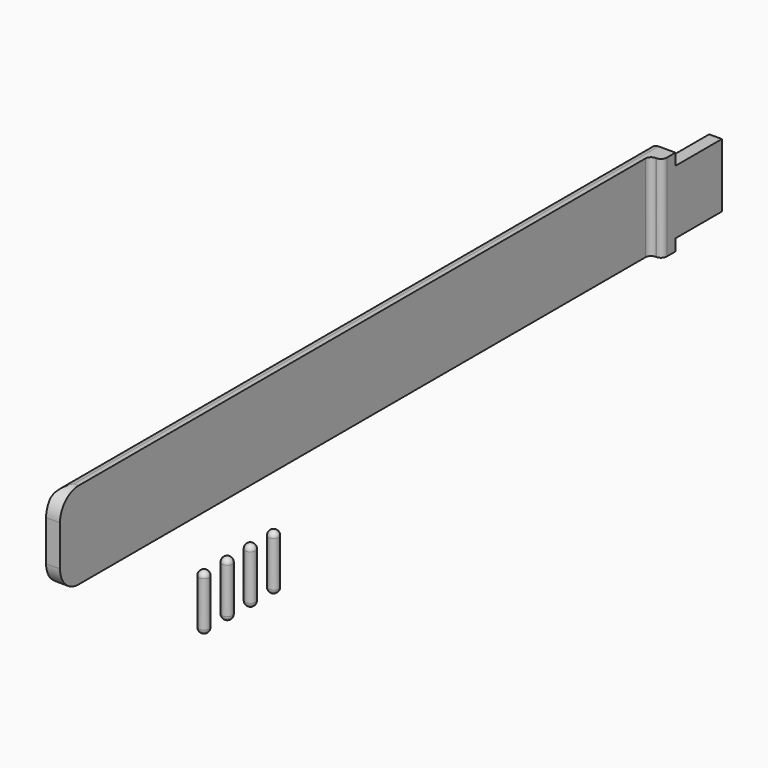
from build123d import *

# Parameters (mm, degrees)
F1_DEPTH    = 19.05
F2_T1_DEPTH = 28.448
F3_T1_DEPTH = 28.448
F4_R        = 1.27
F5_T1_DEPTH = 170.18
F6_W        = 12.7
F6_H        = 2.54
F7_DEPTH    = 25.4
F8_W        = 12.7
F8_H        = 2.54
F9_DEPTH    = 25.4
F10_R       = 1.143
F11_DEPTH   = 12.192
F12_R       = 1.143
F12_2_R     = 1.143
F12_3_R     = 1.143
F12_4_R     = 1.143


# Not quite as in the source:
# - a fillet or chamfer that OpenCascade refuses, or shapes differently, is made with other operations: its cross-section is extruded or revolved along the edge and cut away or added


with BuildPart() as f1:
    # F0 (on Top) → F1 (new body)
    with BuildSketch(Plane.XY):
        Polygon((0, 165.1), (0, 0), (3.048, 0), (3.048, 161.4486724138), (5.715, 161.4486724138), (5.715, 177.8), (2.921, 177.8), (2.921, 165.1), align=None)
    extrude(amount=F1_DEPTH)

    # F2: fillet of radius 5.08 on 1 edges, made by hand

    # F2_s2 → F2_t1 (cut)
    with BuildSketch(Plane.YZ.offset(-12.7)):
        with BuildLine():
            ThreePointArc((0, 13.97), (1.4878975516, 17.5621024484), (5.08, 19.05))
            Line((5.08, 19.05), (0, 19.05))
            Line((0, 19.05), (0, 13.97))
        make_face()
    extrude(amount=F2_T1_DEPTH, mode=Mode.SUBTRACT)

    # F3: fillet of radius 5.08 on 1 edges, made by hand

    # F3_s2 → F3_t1 (cut)
    with BuildSketch(Plane.YZ.offset(-12.7)):
        with BuildLine():
            ThreePointArc((5.08, 0), (1.4878975516, 1.4878975516), (0, 5.08))
            Line((0, 5.08), (0, 0))
            Line((0, 0), (5.08, 0))
        make_face()
    extrude(amount=F3_T1_DEPTH, mode=Mode.SUBTRACT)

    # F4
    f4_edges = [f1.edges().sort_by_distance(p)[0] for p in [
        (5.715, 161.448672, 9.525),
        (3.048, 161.448672, 9.525),
    ]]
    fillet(f4_edges, radius=F4_R)

    # F5: fillet of radius 2.032 on 2 edges, made by hand

    # F5_s2 → F5_t1 (cut)
    with BuildSketch(Plane.XZ.offset(-170.18)):
        with BuildLine():
            ThreePointArc((0, 17.018), (0.5951590206, 18.4548409794), (2.032, 19.05))
            Line((2.032, 19.05), (0, 19.05))
            Line((0, 19.05), (0, 17.018))
        make_face()
        with BuildLine():
            ThreePointArc((2.032, 0), (0.5951590206, 0.5951590206), (0, 2.032))
            Line((0, 2.032), (0, 0))
            Line((0, 0), (2.032, 0))
        make_face()
    extrude(amount=F5_T1_DEPTH, mode=Mode.SUBTRACT)

    # F6 (on face) → F7 (cut)
    with BuildSketch(Plane.YZ.offset(5.715)):
        with Locations((171.45, 17.78)):
            Rectangle(F6_W, F6_H)
    extrude(amount=-F7_DEPTH, mode=Mode.SUBTRACT)

    # F8 (on face) → F9 (cut)
    with BuildSketch(Plane.YZ.offset(5.715)):
        with Locations((171.45, 1.27)):
            Rectangle(F8_W, F8_H)
    extrude(amount=-F9_DEPTH, mode=Mode.SUBTRACT)


with BuildPart() as f11:
    # F10 (on Top) → F11 (new body)
    with BuildSketch(Plane.XY):
        with Locations((30.9944972396, 4.4588609599)):
            Circle(F10_R)
    extrude(amount=F11_DEPTH)

    # F12
    f12_edges = [f11.edges().sort_by_distance(p)[0] for p in [
        (29.851497, 4.458861, 12.192),
        (29.851497, 4.458861, 0),
    ]]
    fillet(f12_edges, radius=F12_R)


with BuildPart() as f11b:
    # F10 (on Top) → F11, piece 2 (new body)
    with BuildSketch(Plane.XY):
        with Locations((30.9944972396, 10.8088609599)):
            Circle(F10_R)
    extrude(amount=F11_DEPTH)

    # F12#2
    f12_2_edges = [f11b.edges().sort_by_distance(p)[0] for p in [
        (29.851497, 10.808861, 12.192),
        (29.851497, 10.808861, 0),
    ]]
    fillet(f12_2_edges, radius=F12_2_R)


with BuildPart() as f11c:
    # F10 (on Top) → F11, piece 3 (new body)
    with BuildSketch(Plane.XY):
        with Locations((30.9944972396, 17.1588609599)):
            Circle(F10_R)
    extrude(amount=F11_DEPTH)

    # F12#3
    f12_3_edges = [f11c.edges().sort_by_distance(p)[0] for p in [
        (29.851497, 17.158861, 12.192),
        (29.851497, 17.158861, 0),
    ]]
    fillet(f12_3_edges, radius=F12_3_R)


with BuildPart() as f11d:
    # F10 (on Top) → F11, piece 4 (new body)
    with BuildSketch(Plane.XY):
        with Locations((30.9944972396, 23.5088609599)):
            Circle(F10_R)
    extrude(amount=F11_DEPTH)

    # F12#4
    f12_4_edges = [f11d.edges().sort_by_distance(p)[0] for p in [
        (29.851497, 23.508861, 12.192),
        (29.851497, 23.508861, 0),
    ]]
    fillet(f12_4_edges, radius=F12_4_R)


solid = Compound([f1.part, f11.part, f11b.part, f11c.part, f11d.part])
